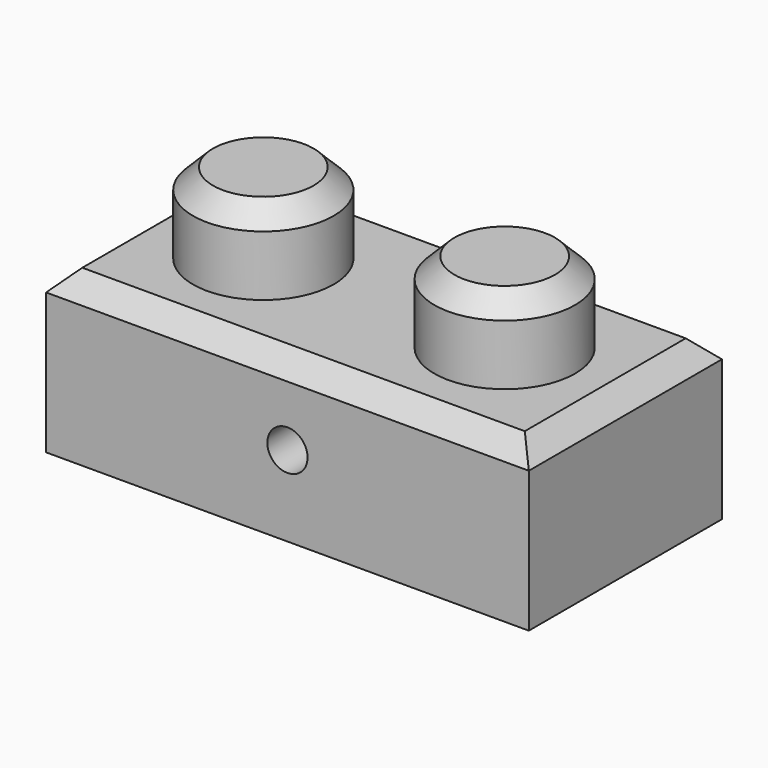
from build123d import *

# Parameters (mm, degrees)
F0_W     = 76.2
F0_H     = 38.1
F1_DEPTH = 25.4
F2_R     = 11.1125
F3_DEPTH = 12.7
F4_SIZE  = 3.175
F5_T     = 7.9375
F6_R     = 3.175
F7_DEPTH = 50.8


# Not quite as in the source:
# - a shell that OpenCascade refuses in one call is made with other operations: the cavity is built on its own and cut out


with BuildPart() as f1:
    # F0 (on Top) → F1 (new body)
    with BuildSketch(Plane.XY):
        with Locations((38.1, 19.05)):
            Rectangle(F0_W, F0_H)
    extrude(amount=F1_DEPTH)

    # F2 (on face) → F3 (join)
    with BuildSketch(Plane.XY.offset(25.4)):
        with Locations((19.05, 19.05)):
            Circle(F2_R)
        with Locations((57.15, 19.05)):
            Circle(F2_R)
    extrude(amount=F3_DEPTH)

    # F4
    f4_edges = [f1.edges().sort_by_distance(p)[0] for p in [
        (7.9375, 19.05, 38.1),
        (0, 19.05, 25.4),
        (38.1, 0, 25.4),
        (76.2, 19.05, 25.4),
        (38.1, 38.1, 25.4),
        (46.0375, 19.05, 38.1),
    ]]
    chamfer(f4_edges, length=F4_SIZE)

    # F5: shell of thickness 7.9375, made by hand


with BuildPart() as f5_core1:
    # F5_t2: copy of F1
    add(f1.part)

    # the walls: a layer under each face that stays
    f5_faces = [f5_core1.faces().sort_by_distance(p)[0] for p in [
        (0, 19.05, 11.1125),
        (38.1, 38.1, 11.1125),
        (1.5875, 19.05, 23.8125),
        (38.1, 0, 11.1125),
        (76.2, 19.05, 11.1125),
        (38.1, 36.5125, 23.8125),
        (38.1, 19.05, 25.4),
        (38.1, 1.5875, 23.8125),
        (74.6125, 19.05, 23.8125),
        (7.9375, 19.05, 30.1625),
        (46.0375, 19.05, 30.1625),
        (9.525, 19.05, 36.5125),
        (47.625, 19.05, 36.5125),
        (19.05, 19.05, 38.1),
        (57.15, 19.05, 38.1),
    ]]
    thicken(f5_faces, amount=-F5_T, mode=Mode.SUBTRACT)

    # F5_s3 → F5_t4 (revolve, cut)
    with BuildSketch(Plane.XZ.offset(-19.05)):
        Polygon((30.241875, 25.479375), (30.1625, 17.4625), (22.225, 17.4625), (22.225, 25.4), align=None)
    revolve(axis=Axis((19.05, 19.05, 25.4), (0, 0, 1)), mode=Mode.SUBTRACT)

    # F5_s5 → F5_t6 (revolve, cut)
    with BuildSketch(Plane.XZ.offset(-19.05)):
        Polygon((68.341875, 25.479375), (68.2625, 17.4625), (60.325, 17.4625), (60.325, 25.4), align=None)
    revolve(axis=Axis((57.15, 19.05, 25.4), (0, 0, 1)), mode=Mode.SUBTRACT)


with BuildPart() as f1_1:
    add(f1.part)

    # what is left inside the walls is the cavity
    f5_cavity = [f5_core1.part.solids().sort_by_distance(p)[0] for p in [
        (38.1, 15.345833, 0.079375),
    ]]
    add(f5_cavity, mode=Mode.SUBTRACT)

    # F6 (on face) → F7 (cut)
    with BuildSketch(Plane.XZ):
        with Locations((38.1, 12.7)):
            Circle(F6_R)
    extrude(amount=-F7_DEPTH, mode=Mode.SUBTRACT)


solid = f1_1.part
